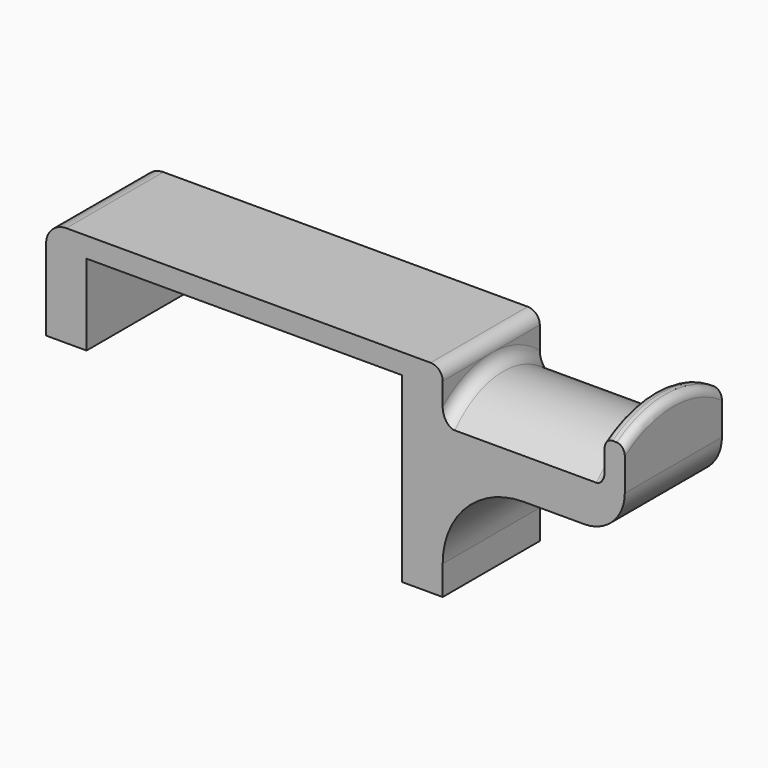
from build123d import *

# Parameters (mm, degrees)
F1_DEPTH = 30
F2_R     = 1
F3_DEPTH = 10
F5_DEPTH = 40
F7_DEPTH = 5
F8_R     = 20
F9_R     = 2.99999
F10_R    = 2
F11_R    = 10
F12_R    = 5


# Not quite as in the source:
# - a fillet or chamfer is up to 0.001 mm smaller than in the source, because OpenCascade refuses the exact size


with BuildPart() as f1:
    # F0 (on Front) → F1 (new body)
    with BuildSketch(Plane.XZ):
        Polygon((0, 45), (0, 0), (10, 0), (10, 50), (-88, 50), (-88, 25), (-78, 25), (-78, 45), align=None)
    extrude(amount=F1_DEPTH)

    # F2 (on face) → F3 (cut, through all)
    with BuildSketch(Plane(origin=(-88, 0, 0), x_dir=(0, -1, 0), z_dir=(-1, 0, 0))):
        with Locations((15, 37.5)):
            Circle(F2_R)
    extrude(amount=-F3_DEPTH, mode=Mode.SUBTRACT)

    # F4 (on face) → F5 (join)
    with BuildSketch(Plane.YZ.offset(10)):
        with BuildLine():
            Line((0, 27.2287565553), (0, 37.2287565553))
            ThreePointArc((0, 37.2287565553), (-15, 44), (-30, 37.2287565553))
            Line((-30, 37.2287565553), (-30, 27.2287565553))
            Line((-30, 27.2287565553), (0, 27.2287565553))
        make_face()
    extrude(amount=F5_DEPTH)

    # F6 (on face) → F7 (join)
    with BuildSketch(Plane.YZ.offset(50)):
        with BuildLine():
            Line((0, 37.2287565553), (0, 47.6431808351))
            ThreePointArc((0, 47.6431808351), (-15, 52), (-30, 47.6431808351))
            Line((-30, 47.6431808351), (-30, 37.2287565553))
            ThreePointArc((-30, 37.2287565553), (-15, 44), (0, 37.2287565553))
        make_face()
        with BuildLine():
            Line((0, 27.2287565553), (0, 37.2287565553))
            ThreePointArc((0, 37.2287565553), (-15, 44), (-30, 37.2287565553))
            Line((-30, 37.2287565553), (-30, 27.2287565553))
            Line((-30, 27.2287565553), (0, 27.2287565553))
        make_face()
    extrude(amount=F7_DEPTH)

    # F8
    f8_edges = [f1.edges().sort_by_distance(p)[0] for p in [
        (10, -15, 27.228757),
    ]]
    fillet(f8_edges, radius=F8_R)

    # F9 (radius 3 in the source; OpenCascade refuses exactly that, so slightly less here)
    f9_edges = [f1.edges().sort_by_distance(p)[0] for p in [
        (10, -15, 44),
        (10, -15, 50),
    ]]
    fillet(f9_edges, radius=F9_R)

    # F10
    f10_edges = [f1.edges().sort_by_distance(p)[0] for p in [
        (50, -15, 44),
        (50, -15, 52),
        (55, -15, 52),
    ]]
    fillet(f10_edges, radius=F10_R)

    # F11
    f11_edges = [f1.edges().sort_by_distance(p)[0] for p in [
        (55, -15, 27.228757),
    ]]
    fillet(f11_edges, radius=F11_R)

    # F12
    f12_edges = [f1.edges().sort_by_distance(p)[0] for p in [
        (-88, -15, 50),
    ]]
    fillet(f12_edges, radius=F12_R)


solid = f1.part
